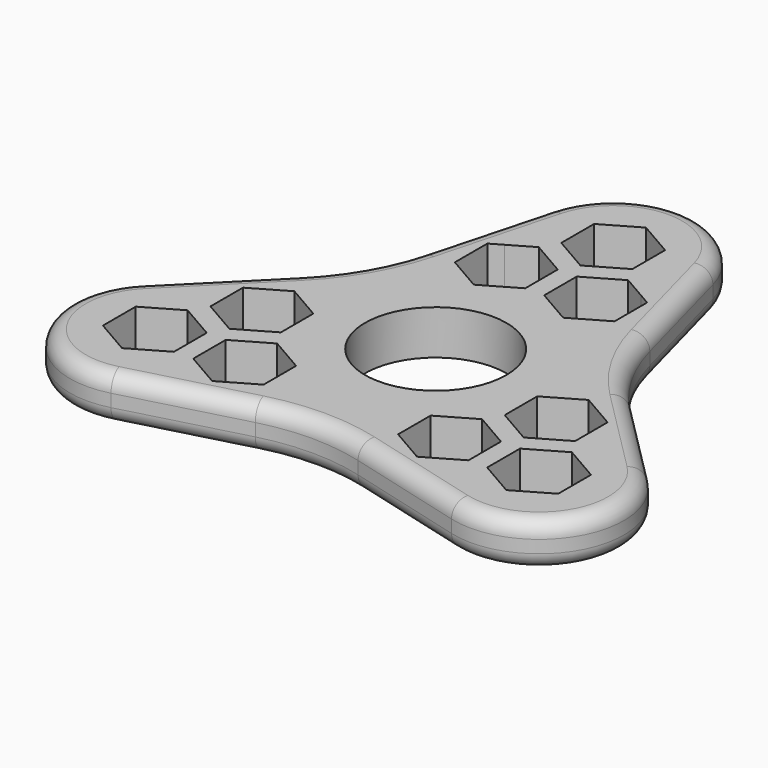
from build123d import *

# Parameters (mm, degrees)
F0_R     = 11.15
F1_DEPTH = 7
F2_R     = 31.4472101729
F3_R     = 2.5


with BuildPart() as f1:
    # F0 (on Top) → F1 (new body)
    with BuildSketch(Plane.XY):
        with BuildLine():
            Line((20.1671623726, 11.6435166246), (12.9445725954, 38.4833765179))
            ThreePointArc((12.9445725954, 38.4833765179), (0, 48.4050688787), (-12.9445725954, 38.4833765179))
            Line((-12.9445725954, 38.4833765179), (-20.1671623726, 11.6435166246))
            Line((-20.1671623726, 11.6435166246), (-39.7998679856, -8.0313595503))
            ThreePointArc((-39.7998679856, -8.0313595503), (-41.9200193209, -24.2025344393), (-26.8552953903, -30.4520169677))
            Line((-26.8552953903, -30.4520169677), (0, -23.2870332492))
            Line((0, -23.2870332492), (26.8552953903, -30.4520169677))
            ThreePointArc((26.8552953903, -30.4520169677), (41.9200193209, -24.2025344393), (39.7998679856, -8.0313595503))
            Line((39.7998679856, -8.0313595503), (20.1671623726, 11.6435166246))
        make_face()
        Polygon((-35.9108891325, -14.2668384925), (-30.3108891325, -11.0336769851), (-24.7108891325, -14.2668384925), (-24.7108891325, -20.7331615075), (-30.3108891325, -23.9663230149), (-35.9108891325, -20.7331615075), align=None, mode=Mode.SUBTRACT)
        Polygon((-16.1608891325, -23.8797204745), (-21.7108891325, -20.6754264805), (-21.7108891325, -14.2668384925), (-16.1608891325, -11.0625444985), (-10.6108891325, -14.2668384925), (-10.6108891325, -20.6754264805), align=None, mode=Mode.SUBTRACT)
        Polygon((-23.2108891325, 1.1484136948), (-17.6608891325, -2.0558802992), (-17.6608891325, -8.4644682872), (-23.2108891325, -11.6687622812), (-28.7608891325, -8.4644682872), (-28.7608891325, -2.0558802992), align=None, mode=Mode.SUBTRACT)
        Polygon((10.6108891325, -20.6754264805), (10.6108891325, -14.2668384925), (16.1608891325, -11.0625444985), (21.7108891325, -14.2668384925), (21.7108891325, -20.6754264805), (16.1608891325, -23.8797204745), align=None, mode=Mode.SUBTRACT)
        Polygon((30.3108891325, -23.9663230149), (24.7108891325, -20.7331615075), (24.7108891325, -14.2668384925), (30.3108891325, -11.0336769851), (35.9108891325, -14.2668384925), (35.9108891325, -20.7331615075), align=None, mode=Mode.SUBTRACT)
        Circle(F0_R, mode=Mode.SUBTRACT)
        Polygon((28.7608891325, -2.0558802992), (28.7608891325, -8.4644682872), (23.2108891325, -11.6687622812), (17.6608891325, -8.4644682872), (17.6608891325, -2.0558802992), (23.2108891325, 1.1484136948), align=None, mode=Mode.SUBTRACT)
        Polygon((-7.05, 29.1398947677), (-1.5, 25.9356007737), (-1.5, 21.6791189615), (-1.5, 19.5270127857), (-7.05, 16.3227187917), (-11.8772290867, 19.1097208044), (-12.6, 19.5270127857), (-12.6, 25.9356007737), (-10.7562631022, 27.000082768), align=None, mode=Mode.SUBTRACT)
        Polygon((10.7562631022, 27.000082768), (12.6, 25.9356007737), (12.6, 19.5270127857), (11.8772290867, 19.1097208044), (7.05, 16.3227187917), (1.5, 19.5270127857), (1.5, 21.6791189615), (1.5, 25.9356007737), (7.05, 29.1398947677), align=None, mode=Mode.SUBTRACT)
        Polygon((0, 41.4663230149), (5.6, 38.2331615075), (5.6, 31.7668384925), (0, 28.5336769851), (-5.6, 31.7668384925), (-5.6, 38.2331615075), align=None, mode=Mode.SUBTRACT)
    extrude(amount=F1_DEPTH)

    # F2
    f2_edges = [f1.edges().sort_by_distance(p)[0] for p in [
        (20.167162, 11.643517, 3.5),
        (-20.167162, 11.643517, 3.5),
        (0, -23.287033, 3.5),
    ]]
    fillet(f2_edges, radius=F2_R)

    # F3
    f3_edges = [f1.edges().sort_by_distance(p)[0] for p in [
        (-32.946681, -1.163452, 7),
        (-21.11979, 12.193517, 0),
    ]]
    fillet(f3_edges, radius=F3_R)


solid = f1.part
